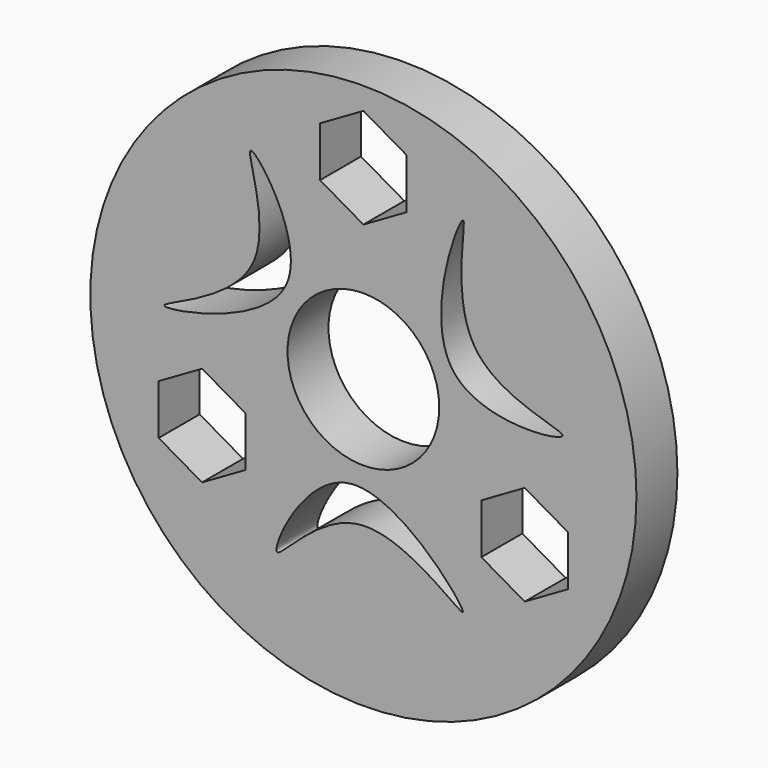
from build123d import *

# Parameters (mm, degrees)
F0_R            = 40
F1_DEPTH        = 7.5
F2_R            = 11.1125
F3_DEPTH        = 25
F5_DEPTH        = 25
F7_DEPTH        = 25
F7_COPIES_COUNT = 3


# Not quite as in the source:
# - a pattern or mirror of a feature is missing from the dataset's text; its kind, count and spacing are read off the source's solid


with BuildPart() as f1:
    # F0 (on Front) → F1 (new body)
    with BuildSketch(Plane.XZ):
        with Locations((0, -2.1214417412)):
            Circle(F0_R)
    extrude(amount=F1_DEPTH)

    # F2 (on face) → F3 (cut)
    with BuildSketch(Plane.XZ.offset(7.5)):
        Circle(F2_R)
    extrude(amount=-F3_DEPTH, mode=Mode.SUBTRACT)

    # F4 (on face) → F5 (cut)
    with BuildSketch(Plane.XZ.offset(7.5)):
        Polygon((6.35, 23.6216606664), (6.35, 30.9540090851), (0, 34.6201832945), (-6.35, 30.9540090851), (-6.35, 23.6216606664), (0, 19.955486457), align=None)
        Polygon((29.9819582167, -17.3100916472), (29.9819582167, -9.9777432285), (23.6319582167, -6.3115690192), (17.2819582167, -9.9777432285), (17.2819582167, -17.3100916472), (23.6319582167, -20.9762658566), align=None)
        Polygon((-17.2819582167, -17.3100916472), (-17.2819582167, -9.9777432285), (-23.6319582167, -6.3115690192), (-29.9819582167, -9.9777432285), (-29.9819582167, -17.3100916472), (-23.6319582167, -20.9762658566), align=None)
    extrude(amount=-F5_DEPTH, mode=Mode.SUBTRACT)

    # F6 (on face) → F7 (cut)
    with BuildSketch(Plane.XZ.offset(7.5)):
        with BuildLine():
            add(Edge.make_bspline(
                [(-29.1492585093, 0), (-28.5084632, -0.5673918386), (-1.1131955523, 4.3103212462), (-21.7557485101, 33.136655751), (-9.1484117303, 6.4453141381), (-29.7266175768, 0.5112222548), (-29.1492585093, 0)],
                knots=[0, 0, 0, 0, 0.2734720596, 0.5207868464, 0.75360061, 1, 1, 1, 1], degree=3))
        make_face()
    f7 = extrude(amount=-F7_DEPTH, mode=Mode.SUBTRACT)

    # F7_copies: F7 ×3 about axis
    f7_copies_axis = Axis((0, 0, 0), (0, 1, 0))
    for i in range(1, F7_COPIES_COUNT):
        add(f7.rotate(f7_copies_axis, i * 360 / F7_COPIES_COUNT), mode=Mode.SUBTRACT)


solid = f1.part
